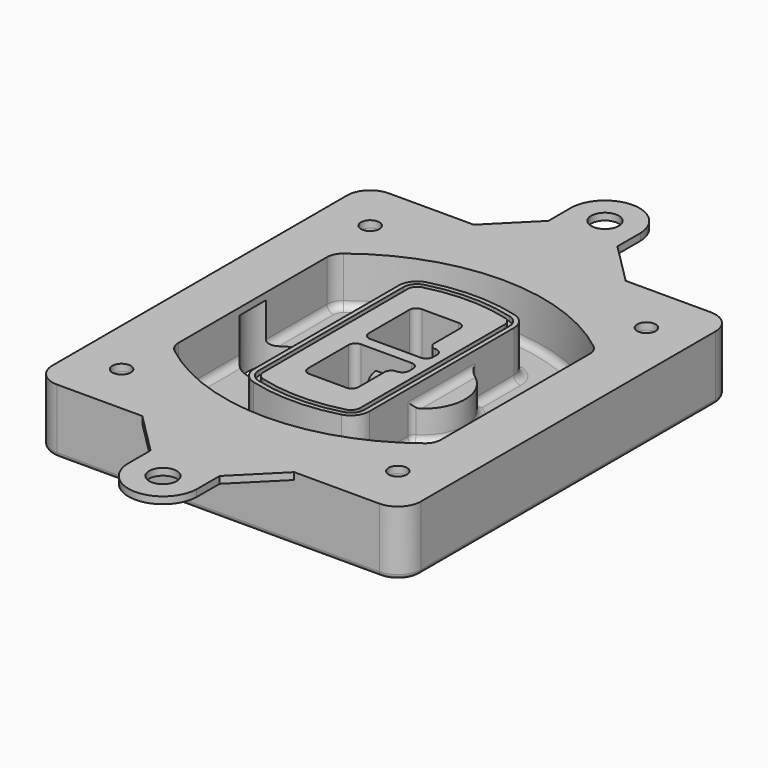
from build123d import *

# Parameters (mm, degrees)
F0_R      = 4
F1_DEPTH  = 25
F2_DEPTH  = 3
F3_DEPTH  = 18
F5_DEPTH  = 21
F6_DEPTH  = 2
F8_DEPTH  = 20
F9_DEPTH  = 16
F10_DEPTH = 25
F7_R      = 6
F7_R_2    = 4
F11_DEPTH = 6
F13_DEPTH = 9
F14_R     = 3
F15_R     = 2
F16_R     = 4
F16_R_2   = 6
F17_DEPTH = 3
F18_DEPTH = 3


# Not quite as in the source:
# - a feature names something its author has since deleted; it is built from what else it names


with BuildPart() as f1:
    # F0 (on Top) → F1 (new body)
    with BuildSketch(Plane.XY):
        with BuildLine():
            ThreePointArc((-80, -80), (-77.0710678119, -87.0710678119), (-70, -90))
            Line((-70, -90), (70, -90))
            ThreePointArc((70, -90), (77.0710678119, -87.0710678119), (80, -80))
            Line((80, -80), (80, 80))
            ThreePointArc((80, 80), (77.0710678119, 87.0710678119), (70, 90))
            Line((70, 90), (-70, 90))
            ThreePointArc((-70, 90), (-77.0710678119, 87.0710678119), (-80, 80))
            Line((-80, 80), (-80, -80))
        make_face()
        with Locations((-60, -67.5)):
            Circle(F0_R, mode=Mode.SUBTRACT)
        with Locations((60, -67.5)):
            Circle(F0_R, mode=Mode.SUBTRACT)
        with Locations((-60, 67.5)):
            Circle(F0_R, mode=Mode.SUBTRACT)
        with BuildLine():
            ThreePointArc((-64, 40.2934422872), (-62.5820384798, 46.4328484224), (-58.6153846154, 51.3286200352))
            ThreePointArc((-58.6153846154, 51.3286200352), (0, 71.5), (58.6153846154, 51.3286200352))
            ThreePointArc((58.6153846154, 51.3286200352), (62.5820384798, 46.4328484224), (64, 40.2934422872))
            Line((64, 40.2934422872), (64, -40.2934422872))
            ThreePointArc((64, -40.2934422872), (62.5820384798, -46.4328484224), (58.6153846154, -51.3286200352))
            ThreePointArc((58.6153846154, -51.3286200352), (0, -71.5), (-58.6153846154, -51.3286200352))
            ThreePointArc((-58.6153846154, -51.3286200352), (-62.5820384798, -46.4328484224), (-64, -40.2934422872))
            Line((-64, -40.2934422872), (-64, 40.2934422872))
        make_face(mode=Mode.SUBTRACT)
        with Locations((60, 67.5)):
            Circle(F0_R, mode=Mode.SUBTRACT)
        with BuildLine():
            ThreePointArc((58.6153846154, 51.3286200352), (0, 71.5), (-58.6153846154, 51.3286200352))
            ThreePointArc((-58.6153846154, 51.3286200352), (-62.5820384798, 46.4328484224), (-64, 40.2934422872))
            Line((-64, 40.2934422872), (-64, -40.2934422872))
            ThreePointArc((-64, -40.2934422872), (-62.5820384798, -46.4328484224), (-58.6153846154, -51.3286200352))
            ThreePointArc((-58.6153846154, -51.3286200352), (0, -71.5), (58.6153846154, -51.3286200352))
            ThreePointArc((58.6153846154, -51.3286200352), (62.5820384798, -46.4328484224), (64, -40.2934422872))
            Line((64, -40.2934422872), (64, 40.2934422872))
            ThreePointArc((64, 40.2934422872), (62.5820384798, 46.4328484224), (58.6153846154, 51.3286200352))
        make_face()
        with BuildLine():
            Line((-60, -40.2934422872), (-60, 40.2934422872))
            ThreePointArc((-60, 40.2934422872), (-58.9871703427, 44.6787323838), (-56.1538461538, 48.1757121072))
            ThreePointArc((-56.1538461538, 48.1757121072), (0, 67.5), (56.1538461538, 48.1757121072))
            ThreePointArc((56.1538461538, 48.1757121072), (58.9871703427, 44.6787323838), (60, 40.2934422872))
            Line((60, 40.2934422872), (60, -40.2934422872))
            ThreePointArc((60, -40.2934422872), (58.9871703427, -44.6787323838), (56.1538461538, -48.1757121072))
            ThreePointArc((56.1538461538, -48.1757121072), (0, -67.5), (-56.1538461538, -48.1757121072))
            ThreePointArc((-56.1538461538, -48.1757121072), (-58.9871703427, -44.6787323838), (-60, -40.2934422872))
        make_face(mode=Mode.SUBTRACT)
        with BuildLine():
            ThreePointArc((-56.1538461538, 48.1757121072), (-58.9871703427, 44.6787323838), (-60, 40.2934422872))
            Line((-60, 40.2934422872), (-60, -40.2934422872))
            ThreePointArc((-60, -40.2934422872), (-58.9871703427, -44.6787323838), (-56.1538461538, -48.1757121072))
            ThreePointArc((-56.1538461538, -48.1757121072), (0, -67.5), (56.1538461538, -48.1757121072))
            ThreePointArc((56.1538461538, -48.1757121072), (58.9871703427, -44.6787323838), (60, -40.2934422872))
            Line((60, -40.2934422872), (60, 40.2934422872))
            ThreePointArc((60, 40.2934422872), (58.9871703427, 44.6787323838), (56.1538461538, 48.1757121072))
            ThreePointArc((56.1538461538, 48.1757121072), (0, 67.5), (-56.1538461538, 48.1757121072))
        make_face()
        with BuildLine():
            ThreePointArc((54.3076923077, 45.8110311612), (56.2910192399, 43.3631453548), (57, 40.2934422872))
            Line((57, 40.2934422872), (57, -40.2934422872))
            ThreePointArc((57, -40.2934422872), (56.2910192399, -43.3631453548), (54.3076923077, -45.8110311612))
            ThreePointArc((54.3076923077, -45.8110311612), (0, -64.5), (-54.3076923077, -45.8110311612))
            ThreePointArc((-54.3076923077, -45.8110311612), (-56.2910192399, -43.3631453548), (-57, -40.2934422872))
            Line((-57, -40.2934422872), (-57, 40.2934422872))
            ThreePointArc((-57, 40.2934422872), (-56.2910192399, 43.3631453548), (-54.3076923077, 45.8110311612))
            ThreePointArc((-54.3076923077, 45.8110311612), (0, 64.5), (54.3076923077, 45.8110311612))
        make_face(mode=Mode.SUBTRACT)
        with BuildLine():
            Line((57, -40.2934422872), (57, 40.2934422872))
            ThreePointArc((57, 40.2934422872), (56.2910192399, 43.3631453548), (54.3076923077, 45.8110311612))
            ThreePointArc((54.3076923077, 45.8110311612), (0, 64.5), (-54.3076923077, 45.8110311612))
            ThreePointArc((-54.3076923077, 45.8110311612), (-56.2910192399, 43.3631453548), (-57, 40.2934422872))
            Line((-57, 40.2934422872), (-57, -40.2934422872))
            ThreePointArc((-57, -40.2934422872), (-56.2910192399, -43.3631453548), (-54.3076923077, -45.8110311612))
            ThreePointArc((-54.3076923077, -45.8110311612), (0, -64.5), (54.3076923077, -45.8110311612))
            ThreePointArc((54.3076923077, -45.8110311612), (56.2910192399, -43.3631453548), (57, -40.2934422872))
        make_face()
    extrude(amount=-F1_DEPTH)

    # F0 (on Top) → F2 (join)
    with BuildSketch(Plane.XY):
        with BuildLine():
            ThreePointArc((-56.1538461538, 48.1757121072), (-58.9871703427, 44.6787323838), (-60, 40.2934422872))
            Line((-60, 40.2934422872), (-60, -40.2934422872))
            ThreePointArc((-60, -40.2934422872), (-58.9871703427, -44.6787323838), (-56.1538461538, -48.1757121072))
            ThreePointArc((-56.1538461538, -48.1757121072), (0, -67.5), (56.1538461538, -48.1757121072))
            ThreePointArc((56.1538461538, -48.1757121072), (58.9871703427, -44.6787323838), (60, -40.2934422872))
            Line((60, -40.2934422872), (60, 40.2934422872))
            ThreePointArc((60, 40.2934422872), (58.9871703427, 44.6787323838), (56.1538461538, 48.1757121072))
            ThreePointArc((56.1538461538, 48.1757121072), (0, 67.5), (-56.1538461538, 48.1757121072))
        make_face()
        with BuildLine():
            ThreePointArc((54.3076923077, 45.8110311612), (56.2910192399, 43.3631453548), (57, 40.2934422872))
            Line((57, 40.2934422872), (57, -40.2934422872))
            ThreePointArc((57, -40.2934422872), (56.2910192399, -43.3631453548), (54.3076923077, -45.8110311612))
            ThreePointArc((54.3076923077, -45.8110311612), (0, -64.5), (-54.3076923077, -45.8110311612))
            ThreePointArc((-54.3076923077, -45.8110311612), (-56.2910192399, -43.3631453548), (-57, -40.2934422872))
            Line((-57, -40.2934422872), (-57, 40.2934422872))
            ThreePointArc((-57, 40.2934422872), (-56.2910192399, 43.3631453548), (-54.3076923077, 45.8110311612))
            ThreePointArc((-54.3076923077, 45.8110311612), (0, 64.5), (54.3076923077, 45.8110311612))
        make_face(mode=Mode.SUBTRACT)
    extrude(amount=F2_DEPTH)

    # F0 (on Top) → F3 (cut)
    with BuildSketch(Plane.XY):
        with BuildLine():
            Line((57, -40.2934422872), (57, 40.2934422872))
            ThreePointArc((57, 40.2934422872), (56.2910192399, 43.3631453548), (54.3076923077, 45.8110311612))
            ThreePointArc((54.3076923077, 45.8110311612), (0, 64.5), (-54.3076923077, 45.8110311612))
            ThreePointArc((-54.3076923077, 45.8110311612), (-56.2910192399, 43.3631453548), (-57, 40.2934422872))
            Line((-57, 40.2934422872), (-57, -40.2934422872))
            ThreePointArc((-57, -40.2934422872), (-56.2910192399, -43.3631453548), (-54.3076923077, -45.8110311612))
            ThreePointArc((-54.3076923077, -45.8110311612), (0, -64.5), (54.3076923077, -45.8110311612))
            ThreePointArc((54.3076923077, -45.8110311612), (56.2910192399, -43.3631453548), (57, -40.2934422872))
        make_face()
    extrude(amount=-F3_DEPTH, mode=Mode.SUBTRACT)

    # F4 (on face) → F5 (join, through all)
    with BuildSketch(Plane.XY.offset(3)):
        with BuildLine():
            ThreePointArc((-25, -39.2465276821), (-23.3511545998, -44.1109737193), (-19.0842911877, -46.9702398883))
            ThreePointArc((-19.0842911877, -46.9702398883), (0, -49.5), (19.0842911877, -46.9702398883))
            ThreePointArc((19.0842911877, -46.9702398883), (23.3511545998, -44.1109737193), (25, -39.2465276821))
            Line((25, -39.2465276821), (25, 39.2465276821))
            ThreePointArc((25, 39.2465276821), (23.3511545998, 44.1109737193), (19.0842911877, 46.9702398883))
            ThreePointArc((19.0842911877, 46.9702398883), (0, 49.5), (-19.0842911877, 46.9702398883))
            ThreePointArc((-19.0842911877, 46.9702398883), (-23.3511545998, 44.1109737193), (-25, 39.2465276821))
            Line((-25, 39.2465276821), (-25, -39.2465276821))
        make_face()
        with BuildLine():
            ThreePointArc((18.5632183908, 45.0393118368), (21.7633659499, 42.89486221), (23, 39.2465276821))
            Line((23, 39.2465276821), (23, -39.2465276821))
            ThreePointArc((23, -39.2465276821), (21.7633659499, -42.89486221), (18.5632183908, -45.0393118368))
            ThreePointArc((18.5632183908, -45.0393118368), (0, -47.5), (-18.5632183908, -45.0393118368))
            ThreePointArc((-18.5632183908, -45.0393118368), (-21.7633659499, -42.89486221), (-23, -39.2465276821))
            Line((-23, -39.2465276821), (-23, 39.2465276821))
            ThreePointArc((-23, 39.2465276821), (-21.7633659499, 42.89486221), (-18.5632183908, 45.0393118368))
            ThreePointArc((-18.5632183908, 45.0393118368), (0, 47.5), (18.5632183908, 45.0393118368))
        make_face(mode=Mode.SUBTRACT)
        with BuildLine():
            Line((23, -39.2465276821), (23, 39.2465276821))
            ThreePointArc((23, 39.2465276821), (21.7633659499, 42.89486221), (18.5632183908, 45.0393118368))
            ThreePointArc((18.5632183908, 45.0393118368), (0, 47.5), (-18.5632183908, 45.0393118368))
            ThreePointArc((-18.5632183908, 45.0393118368), (-21.7633659499, 42.89486221), (-23, 39.2465276821))
            Line((-23, 39.2465276821), (-23, -39.2465276821))
            ThreePointArc((-23, -39.2465276821), (-21.7633659499, -42.89486221), (-18.5632183908, -45.0393118368))
            ThreePointArc((-18.5632183908, -45.0393118368), (0, -47.5), (18.5632183908, -45.0393118368))
            ThreePointArc((18.5632183908, -45.0393118368), (21.7633659499, -42.89486221), (23, -39.2465276821))
        make_face()
        with BuildLine():
            ThreePointArc((18.0421455939, 43.1083837852), (20.1755772999, 41.6787507007), (21, 39.2465276821))
            Line((21, 39.2465276821), (21, -39.2465276821))
            ThreePointArc((21, -39.2465276821), (20.1755772999, -41.6787507007), (18.0421455939, -43.1083837852))
            ThreePointArc((18.0421455939, -43.1083837852), (0, -45.5), (-18.0421455939, -43.1083837852))
            ThreePointArc((-18.0421455939, -43.1083837852), (-20.1755772999, -41.6787507007), (-21, -39.2465276821))
            Line((-21, -39.2465276821), (-21, 39.2465276821))
            ThreePointArc((-21, 39.2465276821), (-20.1755772999, 41.6787507007), (-18.0421455939, 43.1083837852))
            ThreePointArc((-18.0421455939, 43.1083837852), (0, 45.5), (18.0421455939, 43.1083837852))
        make_face(mode=Mode.SUBTRACT)
        with BuildLine():
            Line((21, -39.2465276821), (21, 39.2465276821))
            ThreePointArc((21, 39.2465276821), (20.1755772999, 41.6787507007), (18.0421455939, 43.1083837852))
            ThreePointArc((18.0421455939, 43.1083837852), (0, 45.5), (-18.0421455939, 43.1083837852))
            ThreePointArc((-18.0421455939, 43.1083837852), (-20.1755772999, 41.6787507007), (-21, 39.2465276821))
            Line((-21, 39.2465276821), (-21, -39.2465276821))
            ThreePointArc((-21, -39.2465276821), (-20.1755772999, -41.6787507007), (-18.0421455939, -43.1083837852))
            ThreePointArc((-18.0421455939, -43.1083837852), (0, -45.5), (18.0421455939, -43.1083837852))
            ThreePointArc((18.0421455939, -43.1083837852), (20.1755772999, -41.6787507007), (21, -39.2465276821))
        make_face()
        with BuildLine():
            Line((-8, -2.5), (14, -2.5))
            ThreePointArc((14, -2.5), (16.1213203436, -3.3786796564), (17, -5.5))
            Line((17, -5.5), (17, -7.5))
            ThreePointArc((17, -7.5), (16.1213203436, -9.6213203436), (14, -10.5))
            ThreePointArc((14, -10.5), (11.8786796564, -11.3786796564), (11, -13.5))
            Line((11, -13.5), (11, -27.5))
            ThreePointArc((11, -27.5), (10.1213203436, -29.6213203436), (8, -30.5))
            Line((8, -30.5), (-8, -30.5))
            ThreePointArc((-8, -30.5), (-10.1213203436, -29.6213203436), (-11, -27.5))
            Line((-11, -27.5), (-11, -5.5))
            ThreePointArc((-11, -5.5), (-10.1213203436, -3.3786796564), (-8, -2.5))
        make_face(mode=Mode.SUBTRACT)
        with BuildLine():
            ThreePointArc((-8, 2.5), (-10.1213203436, 3.3786796564), (-11, 5.5))
            Line((-11, 5.5), (-11, 27.5))
            ThreePointArc((-11, 27.5), (-10.1213203436, 29.6213203436), (-8, 30.5))
            Line((-8, 30.5), (8, 30.5))
            ThreePointArc((8, 30.5), (10.1213203436, 29.6213203436), (11, 27.5))
            Line((11, 27.5), (11, 13.5))
            ThreePointArc((11, 13.5), (11.8786796564, 11.3786796564), (14, 10.5))
            ThreePointArc((14, 10.5), (16.1213203436, 9.6213203436), (17, 7.5))
            Line((17, 7.5), (17, 5.5))
            ThreePointArc((17, 5.5), (16.1213203436, 3.3786796564), (14, 2.5))
            Line((14, 2.5), (-8, 2.5))
        make_face(mode=Mode.SUBTRACT)
    extrude(amount=-F5_DEPTH)

    # F4 (on face) → F6 (cut)
    with BuildSketch(Plane.XY.offset(3)):
        with BuildLine():
            Line((23, -39.2465276821), (23, 39.2465276821))
            ThreePointArc((23, 39.2465276821), (21.7633659499, 42.89486221), (18.5632183908, 45.0393118368))
            ThreePointArc((18.5632183908, 45.0393118368), (0, 47.5), (-18.5632183908, 45.0393118368))
            ThreePointArc((-18.5632183908, 45.0393118368), (-21.7633659499, 42.89486221), (-23, 39.2465276821))
            Line((-23, 39.2465276821), (-23, -39.2465276821))
            ThreePointArc((-23, -39.2465276821), (-21.7633659499, -42.89486221), (-18.5632183908, -45.0393118368))
            ThreePointArc((-18.5632183908, -45.0393118368), (0, -47.5), (18.5632183908, -45.0393118368))
            ThreePointArc((18.5632183908, -45.0393118368), (21.7633659499, -42.89486221), (23, -39.2465276821))
        make_face()
        with BuildLine():
            ThreePointArc((18.0421455939, 43.1083837852), (20.1755772999, 41.6787507007), (21, 39.2465276821))
            Line((21, 39.2465276821), (21, -39.2465276821))
            ThreePointArc((21, -39.2465276821), (20.1755772999, -41.6787507007), (18.0421455939, -43.1083837852))
            ThreePointArc((18.0421455939, -43.1083837852), (0, -45.5), (-18.0421455939, -43.1083837852))
            ThreePointArc((-18.0421455939, -43.1083837852), (-20.1755772999, -41.6787507007), (-21, -39.2465276821))
            Line((-21, -39.2465276821), (-21, 39.2465276821))
            ThreePointArc((-21, 39.2465276821), (-20.1755772999, 41.6787507007), (-18.0421455939, 43.1083837852))
            ThreePointArc((-18.0421455939, 43.1083837852), (0, 45.5), (18.0421455939, 43.1083837852))
        make_face(mode=Mode.SUBTRACT)
    extrude(amount=-F6_DEPTH, mode=Mode.SUBTRACT)

    # F7 (on face) → F8 (join)
    with BuildSketch(Plane(origin=(0, 0, -25), x_dir=(1, 0, 0), z_dir=(0, 0, -1))):
        with BuildLine():
            ThreePointArc((3.28842436, 0), (16.7567035675, 13.4682792075), (30.224982775, 0))
            Line((30.224982775, 0), (35.224982775, 0))
            ThreePointArc((35.224982775, 0), (16.7567035675, 18.4682792075), (-1.71157564, 0))
            Line((-1.71157564, 0), (3.28842436, 0))
        make_face()
        with BuildLine():
            Line((3.28842436, 0), (30.224982775, 0))
            ThreePointArc((30.224982775, 0), (16.7567035675, 13.4682792075), (3.28842436, 0))
        make_face()
        with BuildLine():
            ThreePointArc((3.28842436, 0), (16.7567035675, -13.4682792075), (30.224982775, 0))
            Line((30.224982775, 0), (3.28842436, 0))
        make_face()
        with BuildLine():
            Line((35.224982775, 0), (30.224982775, 0))
            ThreePointArc((30.224982775, 0), (16.7567035675, -13.4682792075), (3.28842436, 0))
            Line((3.28842436, 0), (-1.71157564, 0))
            ThreePointArc((-1.71157564, 0), (16.7567035675, -18.4682792075), (35.224982775, 0))
        make_face()
    extrude(amount=-F8_DEPTH)

    # F7 (on face) → F9 (cut)
    with BuildSketch(Plane(origin=(0, 0, -25), x_dir=(1, 0, 0), z_dir=(0, 0, -1))):
        with BuildLine():
            Line((3.28842436, 0), (30.224982775, 0))
            ThreePointArc((30.224982775, 0), (16.7567035675, 13.4682792075), (3.28842436, 0))
        make_face()
        with BuildLine():
            ThreePointArc((3.28842436, 0), (16.7567035675, -13.4682792075), (30.224982775, 0))
            Line((30.224982775, 0), (3.28842436, 0))
        make_face()
    extrude(amount=-F9_DEPTH, mode=Mode.SUBTRACT)

    # F7 (on face) → F10 (cut)
    with BuildSketch(Plane(origin=(0, 0, -25), x_dir=(1, 0, 0), z_dir=(0, 0, -1))):
        with BuildLine():
            Line((-59.0318229325, 0), (-32.0952645175, 0))
            ThreePointArc((-32.0952645175, 0), (-45.563543725, 13.4682792075), (-59.0318229325, 0))
        make_face()
        with BuildLine():
            ThreePointArc((-59.0318229325, 0), (-45.563543725, -13.4682792075), (-32.0952645175, 0))
            Line((-32.0952645175, 0), (-59.0318229325, 0))
        make_face()
    extrude(amount=-F10_DEPTH, mode=Mode.SUBTRACT)

    # F7 (on face) → F11 (cut)
    with BuildSketch(Plane(origin=(0, 0, -25), x_dir=(1, 0, 0), z_dir=(0, 0, -1))):
        with Locations((60, -67.5)):
            Circle(F7_R)
        with Locations((60, -67.5)):
            Circle(F7_R_2, mode=Mode.SUBTRACT)
        with Locations((-60, -67.5)):
            Circle(F7_R)
        with Locations((-60, -67.5)):
            Circle(F7_R_2, mode=Mode.SUBTRACT)
        with Locations((-60, 67.5)):
            Circle(F7_R)
        with Locations((-60, 67.5)):
            Circle(F7_R_2, mode=Mode.SUBTRACT)
        with Locations((60, 67.5)):
            Circle(F7_R)
        with Locations((60, 67.5)):
            Circle(F7_R_2, mode=Mode.SUBTRACT)
    extrude(amount=-F11_DEPTH, mode=Mode.SUBTRACT)

    # F12 (on face) → F13 (cut, through all)
    with BuildSketch(Plane(origin=(0, 0, -9), x_dir=(1, 0, 0), z_dir=(0, 0, -1))):
        with BuildLine():
            Line((11, 13.5), (11, 17.5481537753))
            ThreePointArc((11, 17.5481537753), (2.5696536419, 11.8239143813), (-1.5415842455, 2.5))
            Line((-1.5415842455, 2.5), (3.5224848595, 2.5))
            ThreePointArc((3.5224848595, 2.5), (6.1857188154, 8.3455872281), (11.2536447004, 12.2927168648))
            ThreePointArc((11.2536447004, 12.2927168648), (11.0640958889, 12.8831798879), (11, 13.5))
        make_face()
        with BuildLine():
            ThreePointArc((11.2536447004, -12.2927168648), (6.1857188154, -8.3455872281), (3.5224848595, -2.5))
            Line((3.5224848595, -2.5), (-1.5415842455, -2.5))
            ThreePointArc((-1.5415842455, -2.5), (2.5696536419, -11.8239143813), (11, -17.5481537753))
            Line((11, -17.5481537753), (11, -13.5))
            ThreePointArc((11, -13.5), (11.0640958889, -12.8831798879), (11.2536447004, -12.2927168648))
        make_face()
        with BuildLine():
            ThreePointArc((11.2536447004, 12.2927168648), (6.1857188154, 8.3455872281), (3.5224848595, 2.5))
            Line((3.5224848595, 2.5), (14, 2.5))
            ThreePointArc((14, 2.5), (16.1213203436, 3.3786796564), (17, 5.5))
            Line((17, 5.5), (17, 7.5))
            ThreePointArc((17, 7.5), (16.1213203436, 9.6213203436), (14, 10.5))
            ThreePointArc((14, 10.5), (12.3601599782, 10.9878446101), (11.2536447004, 12.2927168648))
        make_face()
        with BuildLine():
            Line((14, -2.5), (3.5224848595, -2.5))
            ThreePointArc((3.5224848595, -2.5), (6.1857188154, -8.3455872281), (11.2536447004, -12.2927168648))
            ThreePointArc((11.2536447004, -12.2927168648), (12.3601599782, -10.9878446101), (14, -10.5))
            ThreePointArc((14, -10.5), (16.1213203436, -9.6213203436), (17, -7.5))
            Line((17, -7.5), (17, -5.5))
            ThreePointArc((17, -5.5), (16.1213203436, -3.3786796564), (14, -2.5))
        make_face()
    extrude(amount=F13_DEPTH, mode=Mode.SUBTRACT)

    # F14
    f14_edges = [f1.edges().sort_by_distance(p)[0] for p in [
        (-57, -23.703476, -18),
        (-57, 23.703476, -18),
        (25, 0, -5),
        (25, 16.526506, -11.5),
        (25, -16.526506, -11.5),
        (25, -27.886517, -18),
        (35.224983, 0, -18),
    ]]
    fillet(f14_edges, radius=F14_R)

    # F15
    f15_edges = [f1.edges().sort_by_distance(p)[0] for p in [
        (0, -90, -25),
    ]]
    fillet(f15_edges, radius=F15_R)

    # F16 (on face) → F17 (join, through all)
    with BuildSketch(Plane.XY):
        with BuildLine():
            Line((70, 90), (32.9915115143, 90))
            Line((32.9915115143, 90), (0, 90))
            Line((0, 90), (-32.9744896533, 90))
            Line((-32.9744896533, 90), (-32.9915115143, 90))
            Line((-32.9915115143, 90), (-70, 90))
            ThreePointArc((-70, 90), (-77.0710678119, 87.0710678119), (-80, 80))
            Line((-80, 80), (-80, -80))
            ThreePointArc((-80, -80), (-77.0710678119, -87.0710678119), (-70, -90))
            Line((-70, -90), (-32.9915115143, -90))
            Line((-32.9915115143, -90), (32.9915115143, -90))
            Line((32.9915115143, -90), (70, -90))
            ThreePointArc((70, -90), (77.0710678119, -87.0710678119), (80, -80))
            Line((80, -80), (80, 80))
            ThreePointArc((80, 80), (77.0710678119, 87.0710678119), (70, 90))
        make_face()
        with Locations((-60, -67.5)):
            Circle(F16_R, mode=Mode.SUBTRACT)
        with Locations((60, -67.5)):
            Circle(F16_R, mode=Mode.SUBTRACT)
        with Locations((-60, 67.5)):
            Circle(F16_R, mode=Mode.SUBTRACT)
        with BuildLine():
            ThreePointArc((-60, 40.2934422872), (-58.9871703427, 44.6787323838), (-56.1538461538, 48.1757121072))
            ThreePointArc((-56.1538461538, 48.1757121072), (0, 67.5), (56.1538461538, 48.1757121072))
            ThreePointArc((56.1538461538, 48.1757121072), (58.9871703427, 44.6787323838), (60, 40.2934422872))
            Line((60, 40.2934422872), (60, -40.2934422872))
            ThreePointArc((60, -40.2934422872), (58.9871703427, -44.6787323838), (56.1538461538, -48.1757121072))
            ThreePointArc((56.1538461538, -48.1757121072), (0, -67.5), (-56.1538461538, -48.1757121072))
            ThreePointArc((-56.1538461538, -48.1757121072), (-58.9871703427, -44.6787323838), (-60, -40.2934422872))
            Line((-60, -40.2934422872), (-60, 40.2934422872))
        make_face(mode=Mode.SUBTRACT)
        with Locations((60, 67.5)):
            Circle(F16_R, mode=Mode.SUBTRACT)
        with BuildLine():
            Line((14.9915115143, -108), (32.9915115143, -90))
            Line((32.9915115143, -90), (-32.9915115143, -90))
            Line((-32.9915115143, -90), (-14.9915115143, -108))
            Line((-14.9915115143, -108), (-14.9915115143, -120.5045617079))
            ThreePointArc((-14.9915115143, -120.5045617079), (0, -135), (14.9915115143, -120.5045617079))
            Line((14.9915115143, -120.5045617079), (14.9915115143, -108))
        make_face()
        with Locations((0, -120)):
            Circle(F16_R_2, mode=Mode.SUBTRACT)
        with BuildLine():
            Line((14.9915115143, 108), (14.9915115143, 120.5045617079))
            ThreePointArc((14.9915115143, 120.5045617079), (0, 135), (-14.9915115143, 120.5045617079))
            Line((-14.9915115143, 120.5045617079), (-14.9915115143, 108))
            Line((-14.9915115143, 108), (-32.9915115143, 90))
            Line((-32.9915115143, 90), (-32.9744896533, 90))
            Line((-32.9744896533, 90), (0, 90))
            Line((0, 90), (32.9915115143, 90))
            Line((32.9915115143, 90), (14.9915115143, 108))
        make_face()
        with Locations((0, 120)):
            Circle(F16_R_2, mode=Mode.SUBTRACT)
    extrude(amount=F17_DEPTH)

    # F16 (on face) → F18 (join, through all)
    with BuildSketch(Plane.XY):
        with BuildLine():
            Line((14.9915115143, 108), (14.9915115143, 120.5045617079))
            ThreePointArc((14.9915115143, 120.5045617079), (0, 135), (-14.9915115143, 120.5045617079))
            Line((-14.9915115143, 120.5045617079), (-14.9915115143, 108))
            Line((-14.9915115143, 108), (-32.9915115143, 90))
            Line((-32.9915115143, 90), (-32.9744896533, 90))
            Line((-32.9744896533, 90), (0, 90))
            Line((0, 90), (32.9915115143, 90))
            Line((32.9915115143, 90), (14.9915115143, 108))
        make_face()
        with Locations((0, 120)):
            Circle(F16_R_2, mode=Mode.SUBTRACT)
        with BuildLine():
            Line((70, 90), (32.9915115143, 90))
            Line((32.9915115143, 90), (0, 90))
            Line((0, 90), (-32.9744896533, 90))
            Line((-32.9744896533, 90), (-32.9915115143, 90))
            Line((-32.9915115143, 90), (-70, 90))
            ThreePointArc((-70, 90), (-77.0710678119, 87.0710678119), (-80, 80))
            Line((-80, 80), (-80, -80))
            ThreePointArc((-80, -80), (-77.0710678119, -87.0710678119), (-70, -90))
            Line((-70, -90), (-32.9915115143, -90))
            Line((-32.9915115143, -90), (32.9915115143, -90))
            Line((32.9915115143, -90), (70, -90))
            ThreePointArc((70, -90), (77.0710678119, -87.0710678119), (80, -80))
            Line((80, -80), (80, 80))
            ThreePointArc((80, 80), (77.0710678119, 87.0710678119), (70, 90))
        make_face()
        with Locations((-60, -67.5)):
            Circle(F16_R, mode=Mode.SUBTRACT)
        with Locations((60, -67.5)):
            Circle(F16_R, mode=Mode.SUBTRACT)
        with Locations((-60, 67.5)):
            Circle(F16_R, mode=Mode.SUBTRACT)
        with BuildLine():
            ThreePointArc((-60, 40.2934422872), (-58.9871703427, 44.6787323838), (-56.1538461538, 48.1757121072))
            ThreePointArc((-56.1538461538, 48.1757121072), (0, 67.5), (56.1538461538, 48.1757121072))
            ThreePointArc((56.1538461538, 48.1757121072), (58.9871703427, 44.6787323838), (60, 40.2934422872))
            Line((60, 40.2934422872), (60, -40.2934422872))
            ThreePointArc((60, -40.2934422872), (58.9871703427, -44.6787323838), (56.1538461538, -48.1757121072))
            ThreePointArc((56.1538461538, -48.1757121072), (0, -67.5), (-56.1538461538, -48.1757121072))
            ThreePointArc((-56.1538461538, -48.1757121072), (-58.9871703427, -44.6787323838), (-60, -40.2934422872))
            Line((-60, -40.2934422872), (-60, 40.2934422872))
        make_face(mode=Mode.SUBTRACT)
        with Locations((60, 67.5)):
            Circle(F16_R, mode=Mode.SUBTRACT)
    extrude(amount=F18_DEPTH)


solid = f1.part
